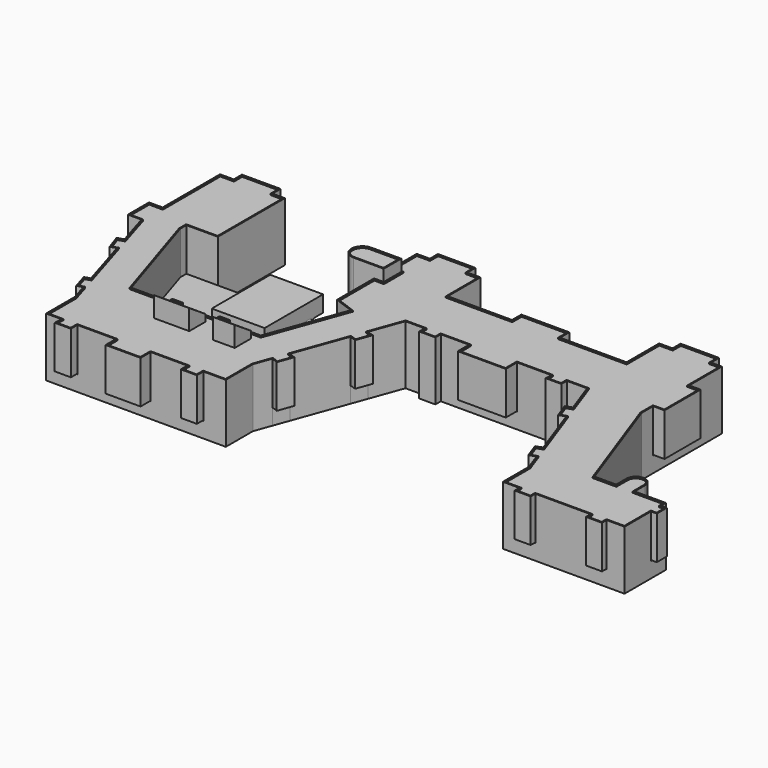
from build123d import *

# Parameters (mm, degrees)
F1_DEPTH      = 12.7
F2_DEPTH      = 15.24
F4_DEPTH      = 0.254
F6_DEPTH      = 0.254
F8_DEPTH      = 3.556
F9_W          = 11.6101317108
F9_H          = 16.0670112818
F10_DEPTH     = 3.556
F11_W         = 32.0663985813
F11_H         = 4.8656136928
F11_W_2       = 25.3707402834
F11_H_2       = 11.204992774
F11_W_3       = 13.6302651196
F11_H_3       = 3.4832812567
F11_W_4       = 1.2735306
F11_H_4       = 6.5489286235
F11_W_5       = 11.4063526
F11_H_5       = 2.2148292
F11_W_6       = 8.2502248
F11_W_7       = 8.5046718858
F11_H_6       = 2.2440223691
F12_DEPTH     = 3.556
F13_R         = 1.27
F14_R         = 0.254
F15_W         = 10.5454804624
F15_H         = 2.5588692216
F16_DEPTH     = 6.35
F18_DEPTH     = 3.556
F19_T1_DEPTH  = 9.911334
F19_T3_DEPTH  = 8.4717128
F19_T5_DEPTH  = 2.7400990862
F19_T7_DEPTH  = 10.5454804624
F19_T9_DEPTH  = 8.2502248
F19_T11_DEPTH = 8.5046718858
F19_T13_DEPTH = 3.5418117158
F19_T15_DEPTH = 3.5439236755
F19_T17_DEPTH = 3.5439236755
F19_T19_DEPTH = 7.6965302
F19_T21_DEPTH = 3.5439236755
F19_T23_DEPTH = 3.5439236755
F19_T25_DEPTH = 3.5439236755
F19_T27_DEPTH = 3.5439236755
F19_T29_DEPTH = 3.5439236755
F19_T34_DEPTH = 17.0410157409
F19_S35_R     = 8.6465238731
F19_T36_DEPTH = 10
F19_T40_DEPTH = 5.8149617531
F19_T45_DEPTH = 5.8149617531
F19_T50_DEPTH = 4.8139236755
F19_T56_DEPTH = 4.8139236755
F21_W         = 4.445
F21_H         = 1.524
F22_DEPTH     = 4.7625
F25_DEPTH     = 7.6965302


# Not quite as in the source:
# - a fillet or chamfer that OpenCascade refuses, or shapes differently, is made with other operations: its cross-section is extruded or revolved along the edge and cut away or added


with BuildPart() as f1:
    # F0 (on Top) → F1 (new body)
    with BuildSketch(Plane.XY):
        with BuildLine():
            Line((11.2178236858, -20.6270437691), (11.2178236858, -2.2440223691))
            Line((11.2178236858, -2.2440223691), (8.5046718858, -2.2440223691))
            Line((8.5046718858, -2.2440223691), (8.5046718858, 0))
            Line((8.5046718858, 0), (0, 0))
            Line((0, 0), (0, -2.2440223691))
            Line((0, -2.2440223691), (-3.0124247142, -2.2440223691))
            Line((-3.0124247142, -2.2440223691), (-3.0124247142, -18.0222062625))
            Line((-3.0124247142, -18.0222062625), (-6.0024365142, -18.0222062625))
            Line((-6.0024365142, -18.0222062625), (-6.0024365142, -23.8371680155))
            Line((-6.0024365142, -23.8371680155), (-3.0124247142, -23.8371680155))
            Line((-3.0124247142, -23.8371680155), (-0.7198106, -31.3397646))
            Line((-0.7198106, -31.3397646), (-2.1268005506, -31.769707085))
            Line((-2.1268005506, -31.769707085), (-0.9747634744, -35.1211553678))
            Line((-0.9747634744, -35.1211553678), (0.3152360415, -34.7269623622))
            Line((0.3152360415, -34.7269623622), (3.840543998, -46.26355863))
            Line((3.840543998, -46.26355863), (2.5818545625, -46.6481840237))
            Line((2.5818545625, -46.6481840237), (3.6175183957, -50.0374015502))
            Line((3.6175183957, -50.0374015502), (4.8762078312, -49.6527761565))
            Line((4.8762078312, -49.6527761565), (5.991627041, -53.3029937409))
            Line((5.991627041, -53.3029937409), (5.991627041, -61.2763585409))
            Line((5.991627041, -61.2763585409), (9.313845441, -61.2763585409))
            Line((9.313845441, -61.2763585409), (9.313845441, -63.0482117409))
            Line((9.313845441, -63.0482117409), (12.8577691165, -63.0482117409))
            Line((12.8577691165, -63.0482117409), (12.8577691165, -61.2763585409))
            Line((12.8577691165, -61.2763585409), (21.273892641, -61.2763585409))
            Line((21.273892641, -61.2763585409), (21.273892641, -64.0449077409))
            Line((21.273892641, -64.0449077409), (28.970422841, -64.0449077409))
            Line((28.970422841, -64.0449077409), (28.970422841, -61.2763585409))
            Line((28.970422841, -61.2763585409), (36.999159641, -61.2763585409))
            Line((36.999159641, -61.2763585409), (36.999159641, -63.0482117409))
            Line((36.999159641, -63.0482117409), (40.5430833165, -63.0482117409))
            Line((40.5430833165, -63.0482117409), (40.5430833165, -61.2763585409))
            Line((40.5430833165, -61.2763585409), (45.483014999, -61.2763585409))
            Line((45.483014999, -61.2763585409), (45.483014999, -53.8215702521))
            Line((45.483014999, -53.8215702521), (46.8170262317, -50.1530457365))
            Line((46.8170262317, -50.1530457365), (48.2096138307, -50.7048616008))
            Line((48.2096138307, -50.7048616008), (49.4207270216, -47.3743061132))
            Line((49.4207270216, -47.3743061132), (48.0281394226, -46.8224902488))
            Line((48.0281394226, -46.8224902488), (52.1718668947, -35.4272595009))
            Line((52.1718668947, -35.4272595009), (53.593629098, -35.8988453429))
            Line((53.593629098, -35.8988453429), (54.8047422888, -32.5682898552))
            Line((54.8047422888, -32.5682898552), (53.3829800855, -32.0967040132))
            Line((53.3829800855, -32.0967040132), (55.9551233498, -25.0233223271))
            Line((55.9551233498, -25.0233223271), (60.1632937498, -25.0233223271))
            Line((60.1632937498, -25.0233223271), (60.1632937498, -26.5212545582))
            Line((60.1632937498, -26.5212545582), (63.7070255498, -26.5212545582))
            Line((63.7070255498, -26.5212545582), (63.7070255498, -25.0233223271))
            Line((63.7070255498, -25.0233223271), (69.9142942606, -25.0233223271))
            Line((69.9142942606, -25.0233223271), (69.9142942606, -28.1078019405))
            Line((69.9142942606, -28.1078019405), (80.459774723, -28.1078019405))
            Line((80.459774723, -28.1078019405), (80.459774723, -25.0233223271))
            Line((80.459774723, -25.0233223271), (87.9593265498, -25.0233223271))
            Line((87.9593265498, -25.0233223271), (87.9593265498, -26.5212545582))
            Line((87.9593265498, -26.5212545582), (91.3923143498, -26.5212545582))
            Line((91.3923143498, -26.5212545582), (91.3923143498, -25.0233223271))
            Line((91.3923143498, -25.0233223271), (95.8516699164, -25.0233223271))
            Line((95.8516699164, -25.0233223271), (98.3801213847, -32.061873401))
            Line((98.3801213847, -32.061873401), (96.970389728, -32.5682898552))
            Line((96.970389728, -32.5682898552), (98.168508858, -35.9035418049))
            Line((98.168508858, -35.9035418049), (99.5782405148, -35.3971253507))
            Line((99.5782405148, -35.3971253507), (103.698871388, -46.867889659))
            Line((103.698871388, -46.867889659), (102.2891397313, -47.3743061132))
            Line((102.2891397313, -47.3743061132), (103.4872588613, -50.7095580628))
            Line((103.4872588613, -50.7095580628), (104.896990518, -50.2031416087))
            Line((104.896990518, -50.2031416087), (106.2471331553, -53.9615874514))
            Line((106.2471331553, -53.9615874514), (106.2471331553, -61.1597696514))
            Line((106.2471331553, -61.1597696514), (109.8462115553, -61.1597696514))
            Line((109.8462115553, -61.1597696514), (109.8462115553, -62.4333002514))
            Line((109.8462115553, -62.4333002514), (113.3901352308, -62.4333002514))
            Line((113.3901352308, -62.4333002514), (113.3901352308, -61.1597696514))
            Line((113.3901352308, -61.1597696514), (125.5160811553, -61.1597696514))
            Line((125.5160811553, -61.1597696514), (125.5160811553, -62.4333002514))
            Line((125.5160811553, -62.4333002514), (129.0600048308, -62.4333002514))
            Line((129.0600048308, -62.4333002514), (129.0600048308, -61.1597696514))
            Line((129.0600048308, -61.1597696514), (132.9911233553, -61.1597696514))
            Line((132.9911233553, -61.1597696514), (132.9911233553, -53.8884918378))
            Line((132.9911233553, -53.8884918378), (134.2646539553, -53.8884918378))
            Line((134.2646539553, -53.8884918378), (134.2646539553, -51.1483927516))
            Line((134.2646539553, -51.1483927516), (132.9911233553, -51.1483927516))
            Line((132.9911233553, -51.1483927516), (132.9911233553, -49.8153018369))
            Line((132.9911233553, -49.8153018369), (126.1268843628, -49.8153018369))
            Line((126.1268843628, -49.8153018369), (126.1268843628, -46.9600556338))
            ThreePointArc((126.1268843628, -46.9600556338), (124.0983568271, -44.9315280982), (122.0698292915, -46.9600556338))
            Line((122.0698292915, -46.9600556338), (122.0698292915, -49.8153018369))
            Line((122.0698292915, -49.8153018369), (117.3079388915, -49.8153018369))
            Line((117.3079388915, -49.8153018369), (108.8542903528, -26.2825436465))
            Line((108.8542903528, -26.2825436465), (108.8542903528, -23.1264158465))
            Line((108.8542903528, -23.1264158465), (111.3459795528, -23.1264158465))
            Line((111.3459795528, -23.1264158465), (111.3459795528, -13.2150818465))
            Line((111.3459795528, -13.2150818465), (108.8542903528, -13.2150818465))
            Line((108.8542903528, -13.2150818465), (108.8542903528, -4.2450464465))
            Line((108.8542903528, -4.2450464465), (106.4733451528, -4.2450464465))
            Line((106.4733451528, -4.2450464465), (106.4733451528, -2.0302172465))
            Line((106.4733451528, -2.0302172465), (98.0016323528, -2.0302172465))
            Line((98.0016323528, -2.0302172465), (98.0016323528, -4.2450464465))
            Line((98.0016323528, -4.2450464465), (95.0669925528, -4.2450464465))
            Line((95.0669925528, -4.2450464465), (95.0669925528, -13.2150818465))
            Line((95.0669925528, -13.2150818465), (80.459774723, -13.2150818465))
            Line((80.459774723, -13.2150818465), (80.459774723, -10.6562126249))
            Line((80.459774723, -10.6562126249), (69.9142942606, -10.6562126249))
            Line((69.9142942606, -10.6562126249), (69.9142942606, -13.2150818465))
            Line((69.9142942606, -13.2150818465), (55.8092605528, -13.2150818465))
            Line((55.8092605528, -13.2150818465), (55.8092605528, -4.2450464465))
            Line((55.8092605528, -4.2450464465), (52.9299927528, -4.2450464465))
            Line((52.9299927528, -4.2450464465), (52.9299927528, -2.0302172465))
            Line((52.9299927528, -2.0302172465), (44.6797679528, -2.0302172465))
            Line((44.6797679528, -2.0302172465), (44.6797679528, -4.2450464465))
            Line((44.6797679528, -4.2450464465), (41.8005001528, -4.2450464465))
            Line((41.8005001528, -4.2450464465), (41.8005001528, -11.1202203191))
            Line((41.8005001528, -11.1202203191), (43.9030276948, -11.1202203191))
            Line((43.9030276948, -11.1202203191), (43.9030276948, -15.9374573191))
            Line((43.9030276948, -15.9374573191), (41.7851103988, -15.9374573191))
            Line((41.7851103988, -15.9374573191), (41.7851103988, -26.1256513191))
            Line((41.7851103988, -26.1256513191), (46.0486273988, -27.6760165191))
            Line((46.0486273988, -27.6760165191), (39.8780233025, -44.6451482986))
            Line((39.8780233025, -44.6451482986), (32.1815185025, -44.6451482986))
            Line((32.1815185025, -44.6451482986), (32.1815185025, -43.4823870986))
            Line((32.1815185025, -43.4823870986), (29.8559453025, -43.4823870986))
            Line((29.8559453025, -43.4823870986), (29.8559453025, -44.6451482986))
            Line((29.8559453025, -44.6451482986), (21.8272085025, -44.6451482986))
            Line((21.8272085025, -44.6451482986), (21.8272085025, -43.4823870986))
            Line((21.8272085025, -43.4823870986), (19.5016353025, -43.4823870986))
            Line((19.5016353025, -43.4823870986), (19.5016353025, -44.6451482986))
            Line((19.5016353025, -44.6451482986), (11.4175519025, -44.6451482986))
            Line((11.4175519025, -44.6451482986), (4.2965014858, -22.2881783691))
            Line((4.2965014858, -22.2881783691), (4.2965014858, -20.6270437691))
            Line((4.2965014858, -20.6270437691), (11.2178236858, -20.6270437691))
        make_face()
        with BuildLine():
            Line((37.3000799988, -15.9374573191), (41.7851103988, -15.9374573191))
            Line((41.7851103988, -15.9374573191), (43.9030276948, -15.9374573191))
            Line((43.9030276948, -15.9374573191), (43.9030276948, -11.1202203191))
            Line((43.9030276948, -11.1202203191), (41.8005001528, -11.1202203191))
            Line((41.8005001528, -11.1202203191), (37.3000799988, -11.1202203191))
            ThreePointArc((37.3000799988, -11.1202203191), (34.8914614988, -13.5288388191), (37.3000799988, -15.9374573191))
        make_face()
    extrude(amount=F1_DEPTH)

    # F0 (on Top) → F2 (join)
    with BuildSketch(Plane.XY):
        with BuildLine():
            Line((37.3000799988, -15.9374573191), (41.7851103988, -15.9374573191))
            Line((41.7851103988, -15.9374573191), (43.9030276948, -15.9374573191))
            Line((43.9030276948, -15.9374573191), (43.9030276948, -11.1202203191))
            Line((43.9030276948, -11.1202203191), (41.8005001528, -11.1202203191))
            Line((41.8005001528, -11.1202203191), (37.3000799988, -11.1202203191))
            ThreePointArc((37.3000799988, -11.1202203191), (34.8914614988, -13.5288388191), (37.3000799988, -15.9374573191))
        make_face()
    extrude(amount=F2_DEPTH)

    # F3 (on face) → F4 (join)
    with BuildSketch(Plane.XY.offset(12.7)):
        with BuildLine():
            Line((53.593629098, -35.8988453429), (54.8047422888, -32.5682898552))
            Line((54.8047422888, -32.5682898552), (53.3829800855, -32.0967040132))
            Line((53.3829800855, -32.0967040132), (55.9551233498, -25.0233223271))
            Line((55.9551233498, -25.0233223271), (60.1632937498, -25.0233223271))
            Line((60.1632937498, -25.0233223271), (60.1632937498, -26.5212545582))
            Line((60.1632937498, -26.5212545582), (63.7070255498, -26.5212545582))
            Line((63.7070255498, -26.5212545582), (63.7070255498, -25.0233223271))
            Line((63.7070255498, -25.0233223271), (69.9142942606, -25.0233223271))
            Line((69.9142942606, -25.0233223271), (69.9142942606, -28.1078019405))
            Line((69.9142942606, -28.1078019405), (80.459774723, -28.1078019405))
            Line((80.459774723, -28.1078019405), (80.459774723, -25.0233223271))
            Line((80.459774723, -25.0233223271), (87.9593265498, -25.0233223271))
            Line((87.9593265498, -25.0233223271), (87.9593265498, -26.5212545582))
            Line((87.9593265498, -26.5212545582), (91.3923143498, -26.5212545582))
            Line((91.3923143498, -26.5212545582), (91.3923143498, -25.0233223271))
            Line((91.3923143498, -25.0233223271), (95.8516699164, -25.0233223271))
            Line((95.8516699164, -25.0233223271), (98.3801213847, -32.061873401))
            Line((98.3801213847, -32.061873401), (96.970389728, -32.5682898552))
            Line((96.970389728, -32.5682898552), (98.168508858, -35.9035418049))
            Line((98.168508858, -35.9035418049), (99.5782405148, -35.3971253507))
            Line((99.5782405148, -35.3971253507), (103.698871388, -46.867889659))
            Line((103.698871388, -46.867889659), (102.2891397313, -47.3743061132))
            Line((102.2891397313, -47.3743061132), (103.4872588613, -50.7095580628))
            Line((103.4872588613, -50.7095580628), (104.896990518, -50.2031416087))
            Line((104.896990518, -50.2031416087), (106.2471331553, -53.9615874514))
            Line((106.2471331553, -53.9615874514), (106.2471331553, -61.1597696514))
            Line((106.2471331553, -61.1597696514), (109.8462115553, -61.1597696514))
            Line((109.8462115553, -61.1597696514), (109.8462115553, -62.4333002514))
            Line((109.8462115553, -62.4333002514), (113.3901352308, -62.4333002514))
            Line((113.3901352308, -62.4333002514), (113.3901352308, -61.1597696514))
            Line((113.3901352308, -61.1597696514), (125.5160811553, -61.1597696514))
            Line((125.5160811553, -61.1597696514), (125.5160811553, -62.4333002514))
            Line((125.5160811553, -62.4333002514), (129.0600048308, -62.4333002514))
            Line((129.0600048308, -62.4333002514), (129.0600048308, -61.1597696514))
            Line((129.0600048308, -61.1597696514), (132.9911233553, -61.1597696514))
            Line((132.9911233553, -61.1597696514), (132.9911233553, -53.8884918378))
            Line((132.9911233553, -53.8884918378), (134.2646539553, -53.8884918378))
            Line((134.2646539553, -53.8884918378), (134.2646539553, -51.1483927516))
            Line((134.2646539553, -51.1483927516), (132.9911233553, -51.1483927516))
            Line((132.9911233553, -51.1483927516), (132.9911233553, -49.8153018369))
            Line((132.9911233553, -49.8153018369), (126.1268843628, -49.8153018369))
            Line((126.1268843628, -49.8153018369), (126.1268843628, -46.9600556338))
            ThreePointArc((126.1268843628, -46.9600556338), (124.0983568271, -44.9315280982), (122.0698292915, -46.9600556338))
            Line((122.0698292915, -46.9600556338), (122.0698292915, -49.8153018369))
            Line((122.0698292915, -49.8153018369), (117.3079388915, -49.8153018369))
            Line((117.3079388915, -49.8153018369), (108.8542903528, -26.2825436465))
            Line((108.8542903528, -26.2825436465), (108.8542903528, -23.1264158465))
            Line((108.8542903528, -23.1264158465), (111.3459795528, -23.1264158465))
            Line((111.3459795528, -23.1264158465), (111.3459795528, -13.2150818465))
            Line((111.3459795528, -13.2150818465), (108.8542903528, -13.2150818465))
            Line((108.8542903528, -13.2150818465), (108.8542903528, -4.2450464465))
            Line((108.8542903528, -4.2450464465), (106.4733451528, -4.2450464465))
            Line((106.4733451528, -4.2450464465), (106.4733451528, -2.0302172465))
            Line((106.4733451528, -2.0302172465), (98.0016323528, -2.0302172465))
            Line((98.0016323528, -2.0302172465), (98.0016323528, -4.2450464465))
            Line((98.0016323528, -4.2450464465), (95.0669925528, -4.2450464465))
            Line((95.0669925528, -4.2450464465), (95.0669925528, -13.2150818465))
            Line((95.0669925528, -13.2150818465), (80.459774723, -13.2150818465))
            Line((80.459774723, -13.2150818465), (80.459774723, -10.6562126249))
            Line((80.459774723, -10.6562126249), (69.9142942606, -10.6562126249))
            Line((69.9142942606, -10.6562126249), (69.9142942606, -13.2150818465))
            Line((69.9142942606, -13.2150818465), (55.8092605528, -13.2150818465))
            Line((55.8092605528, -13.2150818465), (55.8092605528, -4.2450464465))
            Line((55.8092605528, -4.2450464465), (52.9299927528, -4.2450464465))
            Line((52.9299927528, -4.2450464465), (52.9299927528, -2.0302172465))
            Line((52.9299927528, -2.0302172465), (44.6797679528, -2.0302172465))
            Line((44.6797679528, -2.0302172465), (44.6797679528, -4.2450464465))
            Line((44.6797679528, -4.2450464465), (41.8005001528, -4.2450464465))
            Line((41.8005001528, -4.2450464465), (41.8005001528, -11.1202203191))
            Line((41.8005001528, -11.1202203191), (43.9030276948, -11.1202203191))
            Line((43.9030276948, -11.1202203191), (43.9030276948, -15.9374573191))
            Line((43.9030276948, -15.9374573191), (41.7851103988, -15.9374573191))
            Line((41.7851103988, -15.9374573191), (41.7851103988, -26.1256513191))
            Line((41.7851103988, -26.1256513191), (46.0486273988, -27.6760165191))
            Line((46.0486273988, -27.6760165191), (39.8780233025, -44.6451482986))
            Line((39.8780233025, -44.6451482986), (32.1815185025, -44.6451482986))
            Line((32.1815185025, -44.6451482986), (32.1815185025, -43.4823870986))
            Line((32.1815185025, -43.4823870986), (29.8559453025, -43.4823870986))
            Line((29.8559453025, -43.4823870986), (29.8559453025, -44.6451482986))
            Line((29.8559453025, -44.6451482986), (21.8272085025, -44.6451482986))
            Line((21.8272085025, -44.6451482986), (21.8272085025, -43.4823870986))
            Line((21.8272085025, -43.4823870986), (19.5016353025, -43.4823870986))
            Line((19.5016353025, -43.4823870986), (19.5016353025, -44.6451482986))
            Line((19.5016353025, -44.6451482986), (11.4175519025, -44.6451482986))
            Line((11.4175519025, -44.6451482986), (4.2965014858, -22.2881783691))
            Line((4.2965014858, -22.2881783691), (4.2965014858, -20.6270437691))
            Line((4.2965014858, -20.6270437691), (11.2178236858, -20.6270437691))
            Line((11.2178236858, -20.6270437691), (11.2178236858, -2.2440223691))
            Line((11.2178236858, -2.2440223691), (8.5046718858, -2.2440223691))
            Line((8.5046718858, -2.2440223691), (8.5046718858, 0))
            Line((8.5046718858, 0), (0, 0))
            Line((0, 0), (0, -2.2440223691))
            Line((0, -2.2440223691), (-3.0124247142, -2.2440223691))
            Line((-3.0124247142, -2.2440223691), (-3.0124247142, -18.0222062625))
            Line((-3.0124247142, -18.0222062625), (-6.0024365142, -18.0222062625))
            Line((-6.0024365142, -18.0222062625), (-6.0024365142, -23.8371680155))
            Line((-6.0024365142, -23.8371680155), (-3.0124247142, -23.8371680155))
            Line((-3.0124247142, -23.8371680155), (-0.7198106, -31.3397646))
            Line((-0.7198106, -31.3397646), (-2.1268005506, -31.769707085))
            Line((-2.1268005506, -31.769707085), (-0.9747634744, -35.1211553678))
            Line((-0.9747634744, -35.1211553678), (0.3152360415, -34.7269623622))
            Line((0.3152360415, -34.7269623622), (3.840543998, -46.26355863))
            Line((3.840543998, -46.26355863), (2.5818545625, -46.6481840237))
            Line((2.5818545625, -46.6481840237), (3.6175183957, -50.0374015502))
            Line((3.6175183957, -50.0374015502), (4.8762078312, -49.6527761565))
            Line((4.8762078312, -49.6527761565), (5.991627041, -53.3029937409))
            Line((5.991627041, -53.3029937409), (5.991627041, -61.2763585409))
            Line((5.991627041, -61.2763585409), (9.313845441, -61.2763585409))
            Line((9.313845441, -61.2763585409), (9.313845441, -63.0482117409))
            Line((9.313845441, -63.0482117409), (12.8577691165, -63.0482117409))
            Line((12.8577691165, -63.0482117409), (12.8577691165, -61.2763585409))
            Line((12.8577691165, -61.2763585409), (21.273892641, -61.2763585409))
            Line((21.273892641, -61.2763585409), (21.273892641, -64.0449077409))
            Line((21.273892641, -64.0449077409), (28.970422841, -64.0449077409))
            Line((28.970422841, -64.0449077409), (28.970422841, -61.2763585409))
            Line((28.970422841, -61.2763585409), (36.999159641, -61.2763585409))
            Line((36.999159641, -61.2763585409), (36.999159641, -63.0482117409))
            Line((36.999159641, -63.0482117409), (40.5430833165, -63.0482117409))
            Line((40.5430833165, -63.0482117409), (40.5430833165, -61.2763585409))
            Line((40.5430833165, -61.2763585409), (45.483014999, -61.2763585409))
            Line((45.483014999, -61.2763585409), (45.483014999, -53.8215702521))
            Line((45.483014999, -53.8215702521), (46.8170262317, -50.1530457365))
            Line((46.8170262317, -50.1530457365), (48.2096138307, -50.7048616008))
            Line((48.2096138307, -50.7048616008), (49.4207270216, -47.3743061132))
            Line((49.4207270216, -47.3743061132), (48.0281394226, -46.8224902488))
            Line((48.0281394226, -46.8224902488), (52.1718668947, -35.4272595009))
            Line((52.1718668947, -35.4272595009), (53.593629098, -35.8988453429))
        make_face()
        with BuildLine():
            Line((42.0545001528, -10.8662203191), (42.0545001528, -4.4990464465))
            Line((42.0545001528, -4.4990464465), (44.9337679528, -4.4990464465))
            Line((44.9337679528, -4.4990464465), (44.9337679528, -2.2842172465))
            Line((44.9337679528, -2.2842172465), (52.6759927528, -2.2842172465))
            Line((52.6759927528, -2.2842172465), (52.6759927528, -4.4990464465))
            Line((52.6759927528, -4.4990464465), (55.5552605528, -4.4990464465))
            Line((55.5552605528, -4.4990464465), (55.5552605528, -13.4690818465))
            Line((55.5552605528, -13.4690818465), (70.1682942606, -13.4690818465))
            Line((70.1682942606, -13.4690818465), (70.1682942606, -10.9102126249))
            Line((70.1682942606, -10.9102126249), (80.205774723, -10.9102126249))
            Line((80.205774723, -10.9102126249), (80.205774723, -13.4690818465))
            Line((80.205774723, -13.4690818465), (95.3209925528, -13.4690818465))
            Line((95.3209925528, -13.4690818465), (95.3209925528, -4.4990464465))
            Line((95.3209925528, -4.4990464465), (98.2556323528, -4.4990464465))
            Line((98.2556323528, -4.4990464465), (98.2556323528, -2.2842172465))
            Line((98.2556323528, -2.2842172465), (106.2193451528, -2.2842172465))
            Line((106.2193451528, -2.2842172465), (106.2193451528, -4.4990464465))
            Line((106.2193451528, -4.4990464465), (108.6002903528, -4.4990464465))
            Line((108.6002903528, -4.4990464465), (108.6002903528, -13.4690818465))
            Line((108.6002903528, -13.4690818465), (111.0919795528, -13.4690818465))
            Line((111.0919795528, -13.4690818465), (111.0919795528, -22.8724158465))
            Line((111.0919795528, -22.8724158465), (108.6002903528, -22.8724158465))
            Line((108.6002903528, -22.8724158465), (108.6002903528, -26.3267818337))
            Line((108.6002903528, -26.3267818337), (117.1292914119, -50.0693018369))
            Line((117.1292914119, -50.0693018369), (122.3238292915, -50.0693018369))
            Line((122.3238292915, -50.0693018369), (122.3238292915, -46.9600556338))
            ThreePointArc((122.3238292915, -46.9600556338), (124.0983568271, -45.1855280982), (125.8728843628, -46.9600556338))
            Line((125.8728843628, -46.9600556338), (125.8728843628, -50.0693018369))
            Line((125.8728843628, -50.0693018369), (132.7371233553, -50.0693018369))
            Line((132.7371233553, -50.0693018369), (132.7371233553, -51.4023927516))
            Line((132.7371233553, -51.4023927516), (134.0106539553, -51.4023927516))
            Line((134.0106539553, -51.4023927516), (134.0106539553, -53.6344918378))
            Line((134.0106539553, -53.6344918378), (132.7371233553, -53.6344918378))
            Line((132.7371233553, -53.6344918378), (132.7371233553, -60.9057696514))
            Line((132.7371233553, -60.9057696514), (128.8060048308, -60.9057696514))
            Line((128.8060048308, -60.9057696514), (128.8060048308, -62.1793002514))
            Line((128.8060048308, -62.1793002514), (125.7700811553, -62.1793002514))
            Line((125.7700811553, -62.1793002514), (125.7700811553, -60.9057696514))
            Line((125.7700811553, -60.9057696514), (113.1361352308, -60.9057696514))
            Line((113.1361352308, -60.9057696514), (113.1361352308, -62.1793002514))
            Line((113.1361352308, -62.1793002514), (110.1002115553, -62.1793002514))
            Line((110.1002115553, -62.1793002514), (110.1002115553, -60.9057696514))
            Line((110.1002115553, -60.9057696514), (106.5011331553, -60.9057696514))
            Line((106.5011331553, -60.9057696514), (106.5011331553, -53.9173492642))
            Line((106.5011331553, -53.9173492642), (105.0501630426, -49.8782259616))
            Line((105.0501630426, -49.8782259616), (103.6404313858, -50.3846424158))
            Line((103.6404313858, -50.3846424158), (102.6140553783, -47.5274786377))
            Line((102.6140553783, -47.5274786377), (104.0237870351, -47.0210621836))
            Line((104.0237870351, -47.0210621836), (99.7314130393, -35.0722097036))
            Line((99.7314130393, -35.0722097036), (98.3216813826, -35.5786261578))
            Line((98.3216813826, -35.5786261578), (97.2953053751, -32.7214623798))
            Line((97.2953053751, -32.7214623798), (98.7050370318, -32.2150459256))
            Line((98.7050370318, -32.2150459256), (96.030317396, -24.7693223271))
            Line((96.030317396, -24.7693223271), (91.1383143498, -24.7693223271))
            Line((91.1383143498, -24.7693223271), (91.1383143498, -26.2672545582))
            Line((91.1383143498, -26.2672545582), (88.2133265498, -26.2672545582))
            Line((88.2133265498, -26.2672545582), (88.2133265498, -24.7693223271))
            Line((88.2133265498, -24.7693223271), (80.205774723, -24.7693223271))
            Line((80.205774723, -24.7693223271), (80.205774723, -27.8538019405))
            Line((80.205774723, -27.8538019405), (70.1682942606, -27.8538019405))
            Line((70.1682942606, -27.8538019405), (70.1682942606, -24.7693223271))
            Line((70.1682942606, -24.7693223271), (63.4530255498, -24.7693223271))
            Line((63.4530255498, -24.7693223271), (63.4530255498, -26.2672545582))
            Line((63.4530255498, -26.2672545582), (60.4172937498, -26.2672545582))
            Line((60.4172937498, -26.2672545582), (60.4172937498, -24.7693223271))
            Line((60.4172937498, -24.7693223271), (55.7772149302, -24.7693223271))
            Line((55.7772149302, -24.7693223271), (53.0549599378, -32.2555105483))
            Line((53.0549599378, -32.2555105483), (54.4767221411, -32.7270963903))
            Line((54.4767221411, -32.7270963903), (53.4392852211, -35.5800429631))
            Line((53.4392852211, -35.5800429631), (52.0175230178, -35.1084571211))
            Line((52.0175230178, -35.1084571211), (47.7050683372, -46.9676868861))
            Line((47.7050683372, -46.9676868861), (49.0976559362, -47.5195027505))
            Line((49.0976559362, -47.5195027505), (48.0602190162, -50.3724493233))
            Line((48.0602190162, -50.3724493233), (46.6676314172, -49.820633459))
            Line((46.6676314172, -49.820633459), (45.229014999, -53.7768217347))
            Line((45.229014999, -53.7768217347), (45.229014999, -61.0223585409))
            Line((45.229014999, -61.0223585409), (40.2890833165, -61.0223585409))
            Line((40.2890833165, -61.0223585409), (40.2890833165, -62.7942117409))
            Line((40.2890833165, -62.7942117409), (37.253159641, -62.7942117409))
            Line((37.253159641, -62.7942117409), (37.253159641, -61.0223585409))
            Line((37.253159641, -61.0223585409), (28.716422841, -61.0223585409))
            Line((28.716422841, -61.0223585409), (28.716422841, -63.7909077409))
            Line((28.716422841, -63.7909077409), (21.527892641, -63.7909077409))
            Line((21.527892641, -63.7909077409), (21.527892641, -61.0223585409))
            Line((21.527892641, -61.0223585409), (12.6037691165, -61.0223585409))
            Line((12.6037691165, -61.0223585409), (12.6037691165, -62.7942117409))
            Line((12.6037691165, -62.7942117409), (9.567845441, -62.7942117409))
            Line((9.567845441, -62.7942117409), (9.567845441, -61.0223585409))
            Line((9.567845441, -61.0223585409), (6.245627041, -61.0223585409))
            Line((6.245627041, -61.0223585409), (6.245627041, -53.2650515433))
            Line((6.245627041, -53.2650515433), (5.0448916666, -49.3356361816))
            Line((5.0448916666, -49.3356361816), (3.7862022312, -49.7202615753))
            Line((3.7862022312, -49.7202615753), (2.8989945374, -46.8168678591))
            Line((2.8989945374, -46.8168678591), (4.1576839729, -46.4322424654))
            Line((4.1576839729, -46.4322424654), (0.4839198769, -34.4098223873))
            Line((0.4839198769, -34.4098223873), (-0.8143247273, -34.8065348948))
            Line((-0.8143247273, -34.8065348948), (-1.8011257938, -31.9357828952))
            Line((-1.8011257938, -31.9357828952), (-0.4026706251, -31.5084484354))
            Line((-0.4026706251, -31.5084484354), (-2.8244468123, -23.5831680155))
            Line((-2.8244468123, -23.5831680155), (-5.7484365142, -23.5831680155))
            Line((-5.7484365142, -23.5831680155), (-5.7484365142, -18.2762062625))
            Line((-5.7484365142, -18.2762062625), (-2.7584247142, -18.2762062625))
            Line((-2.7584247142, -18.2762062625), (-2.7584247142, -2.4980223691))
            Line((-2.7584247142, -2.4980223691), (0.254, -2.4980223691))
            Line((0.254, -2.4980223691), (0.254, -0.254))
            Line((0.254, -0.254), (8.2506718858, -0.254))
            Line((8.2506718858, -0.254), (8.2506718858, -2.4980223691))
            Line((8.2506718858, -2.4980223691), (10.9638236858, -2.4980223691))
            Line((10.9638236858, -2.4980223691), (10.9638236858, -20.3730437691))
            Line((10.9638236858, -20.3730437691), (4.0425014858, -20.3730437691))
            Line((4.0425014858, -20.3730437691), (4.0425014858, -22.3276528745))
            Line((4.0425014858, -22.3276528745), (11.2318816836, -44.8991482986))
            Line((11.2318816836, -44.8991482986), (19.7556353025, -44.8991482986))
            Line((19.7556353025, -44.8991482986), (19.7556353025, -43.7363870986))
            Line((19.7556353025, -43.7363870986), (21.5732085025, -43.7363870986))
            Line((21.5732085025, -43.7363870986), (21.5732085025, -44.8991482986))
            Line((21.5732085025, -44.8991482986), (30.1099453025, -44.8991482986))
            Line((30.1099453025, -44.8991482986), (30.1099453025, -43.7363870986))
            Line((30.1099453025, -43.7363870986), (31.9275185025, -43.7363870986))
            Line((31.9275185025, -43.7363870986), (31.9275185025, -44.8991482986))
            Line((31.9275185025, -44.8991482986), (40.055931722, -44.8991482986))
            Line((40.055931722, -44.8991482986), (46.3741378827, -27.5241115476))
            Line((46.3741378827, -27.5241115476), (42.0391103988, -25.9477426128))
            Line((42.0391103988, -25.9477426128), (42.0391103988, -16.1914573191))
            Line((42.0391103988, -16.1914573191), (44.1570276948, -16.1914573191))
            Line((44.1570276948, -16.1914573191), (44.1570276948, -10.8662203191))
            Line((44.1570276948, -10.8662203191), (42.0545001528, -10.8662203191))
        make_face(mode=Mode.SUBTRACT)
    extrude(amount=F4_DEPTH)

    # F5 (on face) → F6 (join)
    with BuildSketch(Plane.XY.offset(15.24)):
        with BuildLine():
            ThreePointArc((37.3000799988, -11.1202203191), (34.8914614988, -13.5288388191), (37.3000799988, -15.9374573191))
            Line((37.3000799988, -15.9374573191), (43.9030276948, -15.9374573191))
            Line((43.9030276948, -15.9374573191), (43.9030276948, -11.1202203191))
            Line((43.9030276948, -11.1202203191), (37.3000799988, -11.1202203191))
        make_face()
        with BuildLine():
            Line((37.3000799988, -11.3742203191), (43.6490276948, -11.3742203191))
            Line((43.6490276948, -11.3742203191), (43.6490276948, -15.6834573191))
            Line((43.6490276948, -15.6834573191), (37.3000799988, -15.6834573191))
            ThreePointArc((37.3000799988, -15.6834573191), (35.1454614988, -13.5288388191), (37.3000799988, -11.3742203191))
        make_face(mode=Mode.SUBTRACT)
    extrude(amount=F6_DEPTH)

    # F7 (on face) → F8 (join)
    with BuildSketch(Plane(origin=(0, 0, 0), x_dir=(1, 0, 0), z_dir=(0, 0, -1))):
        Polygon((4.2965014858, 22.2881783691), (4.2965014858, 20.6270437691), (11.2178236858, 20.6270437691), (41.7851103988, 20.6270437691), (41.7851103988, 26.1256513191), (46.0486273988, 27.6760165191), (39.8780233025, 44.6451482986), (32.1815185025, 44.6451482986), (32.1815185025, 43.4823870986), (29.8559453025, 43.4823870986), (29.8559453025, 44.6451482986), (21.8272085025, 44.6451482986), (21.8272085025, 43.4823870986), (19.5016353025, 43.4823870986), (19.5016353025, 44.6451482986), (11.4175519025, 44.6451482986), align=None)
    extrude(amount=-F8_DEPTH)

    # F9 (on face) → F10 (join)
    with BuildSketch(Plane.XY.offset(3.556)):
        with Locations((25.8415769025, -25.2996971831)):
            Rectangle(F9_W, F9_H)
    extrude(amount=F10_DEPTH)

    # F11 (on face) → F12 (cut)
    with BuildSketch(Plane(origin=(0, 0, 0), x_dir=(1, 0, 0), z_dir=(0, 0, -1))):
        with Locations((25.3470447317, 63.7091653873)):
            Rectangle(F11_W, F11_H)
        with Locations((120.732042497, 66.7622660384)):
            Rectangle(F11_W_2, F11_H_2)
        Polygon((-1.6551658009, 28.278807812), (5.4339174361, 51.4778849487), (1.6168511994, 52.1150109378), (-10.073925945, 37.619425824), align=None)
        with Locations((73.6446421632, 26.7649629555)):
            Rectangle(F11_W_3, F11_H_3)
        Polygon((46.1154545423, 52.08236453), (54.2495642123, 29.7136018053), (97.4926848454, 29.5914809552), (105.5720618367, 52.08236453), align=None)
        with Locations((133.6278886553, 50.6140275261)):
            Rectangle(F11_W_4, F11_H_4)
        with Locations((100.7701688528, 3.1376318465)):
            Rectangle(F11_W_5, F11_H_5)
        with Locations((48.8048803528, 3.1376318465)):
            Rectangle(F11_W_6, F11_H_5)
        with Locations((4.2523359429, 1.1220111846)):
            Rectangle(F11_W_7, F11_H_6)
        Polygon((114.0086125186, 25.9879335358), (108.8542903528, 23.1264158465), (108.8542903528, 13.2150818465), (112.9228579967, 10.0683534115), align=None)
        Polygon((-7.6378895901, 16.1495096982), (-3.0124247142, 18.0222062625), (-3.0124247142, 23.8371680155), (-9.3068471178, 26.7690140754), align=None)
    extrude(amount=-F12_DEPTH, mode=Mode.SUBTRACT)

    # F13
    f13_edges = [f1.edges().sort_by_distance(p)[0] for p in [
        (25.841577, -20.627044, 3.556),
    ]]
    fillet(f13_edges, radius=F13_R)

    # F14
    f14_edges = [f1.edges().sort_by_distance(p)[0] for p in [
        (20.036511, -26.980123, 3.556),
        (25.841577, -33.333203, 3.556),
        (31.646643, -26.980123, 3.556),
    ]]
    fillet(f14_edges, radius=F14_R)

    # F15 (on face) → F16 (cut)
    with BuildSketch(Plane(origin=(0, 0, 0), x_dir=(1, 0, 0), z_dir=(0, 0, -1))):
        with Locations((75.1870344918, 11.9356472357)):
            Rectangle(F15_W, F15_H)
    extrude(amount=-F16_DEPTH, mode=Mode.SUBTRACT)

    # F17 (on face) → F18 (join)
    with BuildSketch(Plane(origin=(0, 0, 0), x_dir=(1, 0, 0), z_dir=(0, 0, -1))):
        with BuildLine():
            Line((83.3236344233, 13.2150818465), (67.5526186824, 13.2150818465))
            ThreePointArc((67.5526186824, 13.2150818465), (75.4381265528, 8.1155483474), (83.3236344233, 13.2150818465))
        make_face()
    extrude(amount=-F18_DEPTH)

    # F19: fillet of radius 0.254 on 20 edges, made by hand

    # F19_s2 → F19_t1 (join)
    with BuildSketch(Plane.XZ.offset(13.2150818465)):
        with BuildLine():
            ThreePointArc((108.8542903528, 3.302), (108.9286852304, 3.4816051224), (109.1082903528, 3.556))
            Line((109.1082903528, 3.556), (108.8542903528, 3.556))
            Line((108.8542903528, 3.556), (108.8542903528, 3.302))
        make_face()
    extrude(amount=F19_T1_DEPTH)

    # F19_s4 → F19_t3 (join)
    with BuildSketch(Plane.YZ.offset(98.0016323528)):
        with BuildLine():
            ThreePointArc((-4.2450464465, 3.302), (-4.1706515689, 3.4816051224), (-3.9910464465, 3.556))
            Line((-3.9910464465, 3.556), (-4.2450464465, 3.556))
            Line((-4.2450464465, 3.556), (-4.2450464465, 3.302))
        make_face()
    extrude(amount=F19_T3_DEPTH)

    # F19_s6 → F19_t5 (join)
    with BuildSketch(Plane.XZ.offset(51.1483927516)):
        with BuildLine():
            ThreePointArc((132.9911233553, 3.302), (133.0655182329, 3.4816051224), (133.2451233553, 3.556))
            Line((133.2451233553, 3.556), (132.9911233553, 3.556))
            Line((132.9911233553, 3.556), (132.9911233553, 3.302))
        make_face()
    extrude(amount=F19_T5_DEPTH)

    # F19_s8 → F19_t7 (join)
    with BuildSketch(Plane.YZ.offset(69.9142942606)):
        with BuildLine():
            ThreePointArc((-13.2150818465, 6.096), (-13.1406869689, 6.2756051224), (-12.9610818465, 6.35))
            Line((-12.9610818465, 6.35), (-13.2150818465, 6.35))
            Line((-13.2150818465, 6.35), (-13.2150818465, 6.096))
        make_face()
        with BuildLine():
            ThreePointArc((-25.0233223271, 3.302), (-25.0977172047, 3.4816051224), (-25.2773223271, 3.556))
            Line((-25.2773223271, 3.556), (-25.0233223271, 3.556))
            Line((-25.0233223271, 3.556), (-25.0233223271, 3.302))
        make_face()
    extrude(amount=F19_T7_DEPTH)

    # F19_s10 → F19_t9 (join)
    with BuildSketch(Plane.YZ.offset(44.6797679528)):
        with BuildLine():
            ThreePointArc((-4.2450464465, 3.302), (-4.1706515689, 3.4816051224), (-3.9910464465, 3.556))
            Line((-3.9910464465, 3.556), (-4.2450464465, 3.556))
            Line((-4.2450464465, 3.556), (-4.2450464465, 3.302))
        make_face()
    extrude(amount=F19_T9_DEPTH)

    # F19_s12 → F19_t11 (join)
    with BuildSketch(Plane.YZ):
        with BuildLine():
            ThreePointArc((-2.2440223691, 3.302), (-2.1696274916, 3.4816051224), (-1.9900223691, 3.556))
            Line((-1.9900223691, 3.556), (-2.2440223691, 3.556))
            Line((-2.2440223691, 3.556), (-2.2440223691, 3.302))
        make_face()
    extrude(amount=F19_T11_DEPTH)

    # F19_s14 → F19_t13 (join)
    with BuildSketch(Plane(origin=(8.6973398081, -28.4621086181, 0), x_dir=(0, 0, 1), z_dir=(0.2922364949, -0.9563460833, 0))):
        with BuildLine():
            ThreePointArc((3.302, 9.8470110064), (3.4816051224, 9.921405884), (3.556, 10.1010110064))
            Line((3.556, 10.1010110064), (3.556, 9.8470110064))
            Line((3.556, 9.8470110064), (3.302, 9.8470110064))
        make_face()
    extrude(amount=F19_T13_DEPTH)

    # F19_s16 → F19_t15 (join)
    with BuildSketch(Plane(origin=(13.2576944061, -43.385902648, 0), x_dir=(0, 0, 1), z_dir=(0.2922364949, -0.9563460833, 0))):
        with BuildLine():
            ThreePointArc((3.302, 9.8470110064), (3.4816051224, 9.921405884), (3.556, 10.1010110064))
            Line((3.556, 10.1010110064), (3.556, 9.8470110064))
            Line((3.556, 9.8470110064), (3.302, 9.8470110064))
        make_face()
    extrude(amount=F19_T15_DEPTH)

    # F19_s18 → F19_t17 (join)
    with BuildSketch(Plane.YZ.offset(9.313845441)):
        with BuildLine():
            ThreePointArc((-61.2763585409, 3.302), (-61.3507534185, 3.4816051224), (-61.5303585409, 3.556))
            Line((-61.5303585409, 3.556), (-61.2763585409, 3.556))
            Line((-61.2763585409, 3.556), (-61.2763585409, 3.302))
        make_face()
    extrude(amount=F19_T17_DEPTH)

    # F19_s20 → F19_t19 (join)
    with BuildSketch(Plane.YZ.offset(21.273892641)):
        with BuildLine():
            ThreePointArc((-61.2763585409, 3.302), (-61.3507534185, 3.4816051224), (-61.5303585409, 3.556))
            Line((-61.5303585409, 3.556), (-61.2763585409, 3.556))
            Line((-61.2763585409, 3.556), (-61.2763585409, 3.302))
        make_face()
    extrude(amount=F19_T19_DEPTH)

    # F19_s22 → F19_t21 (join)
    with BuildSketch(Plane.YZ.offset(36.999159641)):
        with BuildLine():
            ThreePointArc((-61.2763585409, 3.302), (-61.3507534185, 3.4816051224), (-61.5303585409, 3.556))
            Line((-61.5303585409, 3.556), (-61.2763585409, 3.556))
            Line((-61.2763585409, 3.556), (-61.2763585409, 3.302))
        make_face()
    extrude(amount=F19_T21_DEPTH)

    # F19_s24 → F19_t23 (join)
    with BuildSketch(Plane.YZ.offset(109.8462115553)):
        with BuildLine():
            ThreePointArc((-61.1597696514, 3.302), (-61.234164529, 3.4816051224), (-61.4137696514, 3.556))
            Line((-61.4137696514, 3.556), (-61.1597696514, 3.556))
            Line((-61.1597696514, 3.556), (-61.1597696514, 3.302))
        make_face()
    extrude(amount=F19_T23_DEPTH)

    # F19_s26 → F19_t25 (join)
    with BuildSketch(Plane.YZ.offset(125.5160811553)):
        with BuildLine():
            ThreePointArc((-61.1597696514, 3.302), (-61.234164529, 3.4816051224), (-61.4137696514, 3.556))
            Line((-61.4137696514, 3.556), (-61.1597696514, 3.556))
            Line((-61.1597696514, 3.556), (-61.1597696514, 3.302))
        make_face()
    extrude(amount=F19_T25_DEPTH)

    # F19_s28 → F19_t27 (join)
    with BuildSketch(Plane(origin=(26.7643536419, -74.5049973984, 0), x_dir=(0, 0, 1), z_dir=(0.3380770129, -0.9411184481, 0))):
        with BuildLine():
            ThreePointArc((3.302, -81.7479647761), (3.4816051224, -81.6735698985), (3.556, -81.4939647761))
            Line((3.556, -81.4939647761), (3.556, -81.7479647761))
            Line((3.556, -81.7479647761), (3.302, -81.7479647761))
        make_face()
    extrude(amount=F19_T27_DEPTH)

    # F19_s30 → F19_t29 (join)
    with BuildSketch(Plane(origin=(21.4456036386, -59.6989811404, 0), x_dir=(0, 0, 1), z_dir=(0.3380770129, -0.9411184481, 0))):
        with BuildLine():
            ThreePointArc((3.302, -81.7479647761), (3.4816051224, -81.6735698985), (3.556, -81.4939647761))
            Line((3.556, -81.4939647761), (3.556, -81.7479647761))
            Line((3.556, -81.7479647761), (3.302, -81.7479647761))
        make_face()
    extrude(amount=F19_T29_DEPTH)


with BuildPart() as f19_tool32:
    # F19_s33 → F19_t34 (new body)
    with BuildSketch(Plane.YZ.offset(83.9586344233)):
        with BuildLine():
            ThreePointArc((-13.2150818465, 3.81), (-13.1406869689, 3.6303948776), (-12.9610818465, 3.556))
            Line((-12.9610818465, 3.556), (-13.2150818465, 3.556))
            Line((-13.2150818465, 3.556), (-13.2150818465, 3.81))
        make_face()
    extrude(amount=-F19_T34_DEPTH)

    # F19_s35 → F19_t36 (intersect, symmetric)
    with BuildSketch(Plane.XY.offset(3.7)):
        with Locations((75.4381265528, -16.7620722204)):
            Circle(F19_S35_R)
    extrude(amount=F19_T36_DEPTH, both=True, mode=Mode.INTERSECT)


with BuildPart() as f1_1:
    add(f1.part)

    # F19_t31: union F19_tool32
    add(f19_tool32.part)


with BuildPart() as f19_tool38:
    # F19_s39 → F19_t40 (new body)
    with BuildSketch(Plane.XZ.offset(18.0222062625)):
        with BuildLine():
            ThreePointArc((-3.0124247142, 3.302), (-3.0868195918, 3.4816051224), (-3.2664247142, 3.556))
            Line((-3.2664247142, 3.556), (-3.0124247142, 3.556))
            Line((-3.0124247142, 3.556), (-3.0124247142, 3.302))
        make_face()
    extrude(amount=F19_T40_DEPTH)

    split(bisect_by=Plane(origin=(-9.4171504081, -2.8776559819, 0), x_dir=(0, 0, 1), z_dir=(0.9563460833, 0.2922364949, 0)), keep=Keep.TOP)


with BuildPart() as f1_2:
    add(f1_1.part)

    # F19_t37: union F19_tool38
    add(f19_tool38.part)


with BuildPart() as f19_tool43:
    # F19_s44 → F19_t45 (new body)
    with BuildSketch(Plane.XZ.offset(18.0222062625)):
        with BuildLine():
            ThreePointArc((-3.0124247142, 3.302), (-3.0868195918, 3.4816051224), (-3.2664247142, 3.556))
            Line((-3.2664247142, 3.556), (-3.0124247142, 3.556))
            Line((-3.0124247142, 3.556), (-3.0124247142, 3.302))
        make_face()
    extrude(amount=F19_T45_DEPTH)

    split(bisect_by=Plane(origin=(-9.4171504081, -2.8776559819, 0), x_dir=(0, 0, 1), z_dir=(-0.9563460833, -0.2922364949, 0)), keep=Keep.TOP)


with BuildPart() as f1_3:
    add(f1_2.part)

    # F19_t42: union F19_tool43
    add(f19_tool43.part)


with BuildPart() as f19_tool48:
    # F19_s49 → F19_t50 (new body)
    with BuildSketch(Plane(origin=(-10.856877487, -29.8563612111, 0), x_dir=(0, 0, 1), z_dir=(0.3417435875, 0.9397932328, 0))):
        with BuildLine():
            ThreePointArc((3.302, 61.1378062077), (3.4816051224, 61.2122010852), (3.556, 61.3918062077))
            Line((3.556, 61.3918062077), (3.556, 61.1378062077))
            Line((3.556, 61.1378062077), (3.302, 61.1378062077))
        make_face()
    extrude(amount=F19_T50_DEPTH)

    split(bisect_by=Plane(origin=(-10.8228784969, -27.3131081466, 0), x_dir=(0, 0, 1), z_dir=(0.3683850664, 0.929673299, 0)), keep=Keep.TOP)

    split(bisect_by=Plane(origin=(-9.5178801016, -24.0197548754, 0), x_dir=(0, 0, 1), z_dir=(-0.3683850664, -0.929673299, 0)), keep=Keep.TOP)


with BuildPart() as f1_4:
    add(f1_3.part)

    # F19_t47: union F19_tool48
    add(f19_tool48.part)


with BuildPart() as f19_tool54:
    # F19_s55 → F19_t56 (new body)
    with BuildSketch(Plane(origin=(-5.5020368241, -15.1305749755, 0), x_dir=(0, 0, 1), z_dir=(0.3417435875, 0.9397932328, 0))):
        with BuildLine():
            ThreePointArc((3.302, 61.1378062077), (3.4816051224, 61.2122010852), (3.556, 61.3918062077))
            Line((3.556, 61.3918062077), (3.556, 61.1378062077))
            Line((3.556, 61.1378062077), (3.302, 61.1378062077))
        make_face()
    extrude(amount=F19_T56_DEPTH)

    split(bisect_by=Plane(origin=(-4.2999713611, -12.9637834981, 0), x_dir=(0, 0, 1), z_dir=(-0.3148245509, -0.9491498839, 0)), keep=Keep.TOP)

    split(bisect_by=Plane(origin=(-5.4152324596, -16.3261322699, 0), x_dir=(0, 0, 1), z_dir=(0.3148245509, 0.9491498839, 0)), keep=Keep.TOP)


with BuildPart() as f1_5:
    add(f1_4.part)

    # F19_t53: union F19_tool54
    add(f19_tool54.part)

    # F24 (on offset) → F25 (join, through all)
    with BuildSketch(Plane.YZ.offset(28.970422841)):
        Polygon((-50.680693993, 17.145), (-50.680693993, 12.7), (-46.235693993, 12.7), (-46.235693993, 14.224), align=None)
    extrude(amount=-F25_DEPTH)


with BuildPart() as f22:
    # F21 (on offset) → F22 (new body)
    with BuildSketch(Plane.YZ.offset(38.9555833165)):
        with Locations((-48.458193993, 13.462)):
            Rectangle(F21_W, F21_H)
        Polygon((-50.680693993, 14.224), (-46.235693993, 14.224), (-50.680693993, 17.145), align=None)
    extrude(amount=-F22_DEPTH)


solid = Compound([f1_5.part, f22.part])
